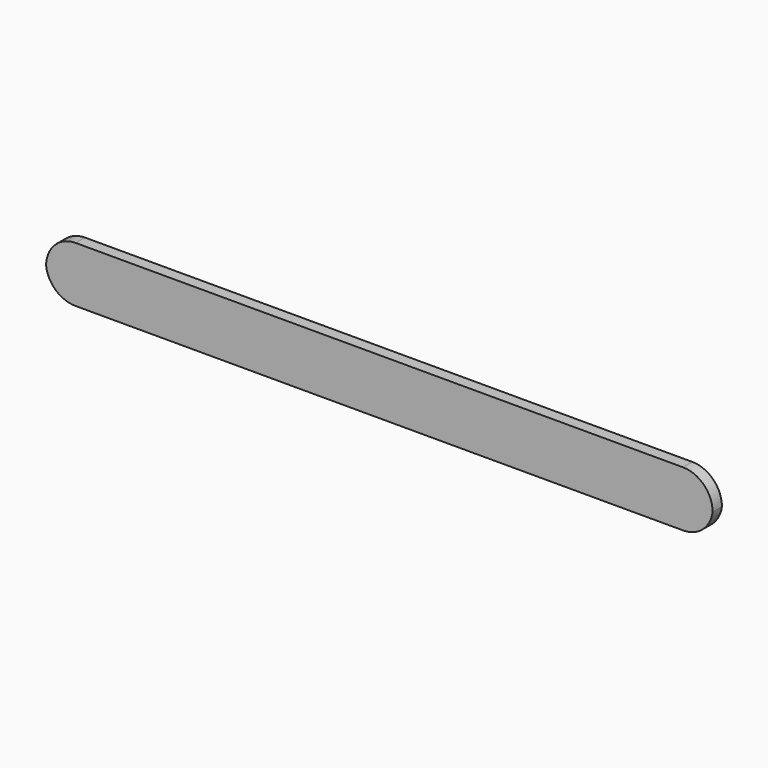
from build123d import *

# Parameters (mm, degrees)
F0_W        = 114.3
F0_H        = 9.525
F1_DEPTH    = 1.99898
F2_R        = 5.08
F3_T1_DEPTH = 27.1997612379
F4_R        = 5.08
F5_T1_DEPTH = 27.1997612379


# Not quite as in the source:
# - a fillet or chamfer that OpenCascade refuses, or shapes differently, is made with other operations: its cross-section is extruded or revolved along the edge and cut away or added


with BuildPart() as f1:
    # F0 (on Front) → F1 (new body)
    with BuildSketch(Plane.XZ):
        with Locations((5.390194959, -14.5571018083)):
            Rectangle(F0_W, F0_H)
    extrude(amount=F1_DEPTH)

    # F2
    f2_edges = [f1.edges().sort_by_distance(p)[0] for p in [
        (-51.759805, -0.99949, -9.794602),
    ]]
    fillet(f2_edges, radius=F2_R)

    # F3: fillet of radius 5.08 on 1 edges, made by hand

    # F3_s2 → F3_t1 (cut)
    with BuildSketch(Plane.XZ.offset(-12.6003906189)):
        with BuildLine():
            ThreePointArc((-51.759805041, -14.8746018083), (-50.0797529584, -18.0496018083), (-46.7196487934, -19.3196018083))
            Line((-46.7196487934, -19.3196018083), (-51.759805041, -19.3196018083))
            Line((-51.759805041, -19.3196018083), (-51.759805041, -14.8746018083))
        make_face()
    extrude(amount=F3_T1_DEPTH, mode=Mode.SUBTRACT)

    # F4
    f4_edges = [f1.edges().sort_by_distance(p)[0] for p in [
        (62.540195, -0.99949, -9.794602),
    ]]
    fillet(f4_edges, radius=F4_R)

    # F5: fillet of radius 5.08 on 1 edges, made by hand

    # F5_s2 → F5_t1 (cut)
    with BuildSketch(Plane.XZ.offset(-12.6003906189)):
        with BuildLine():
            ThreePointArc((62.540194959, -14.8746018083), (60.8601428765, -18.0496018083), (57.5000387115, -19.3196018083))
            Line((57.5000387115, -19.3196018083), (62.540194959, -19.3196018083))
            Line((62.540194959, -19.3196018083), (62.540194959, -14.8746018083))
        make_face()
    extrude(amount=F5_T1_DEPTH, mode=Mode.SUBTRACT)


solid = f1.part
